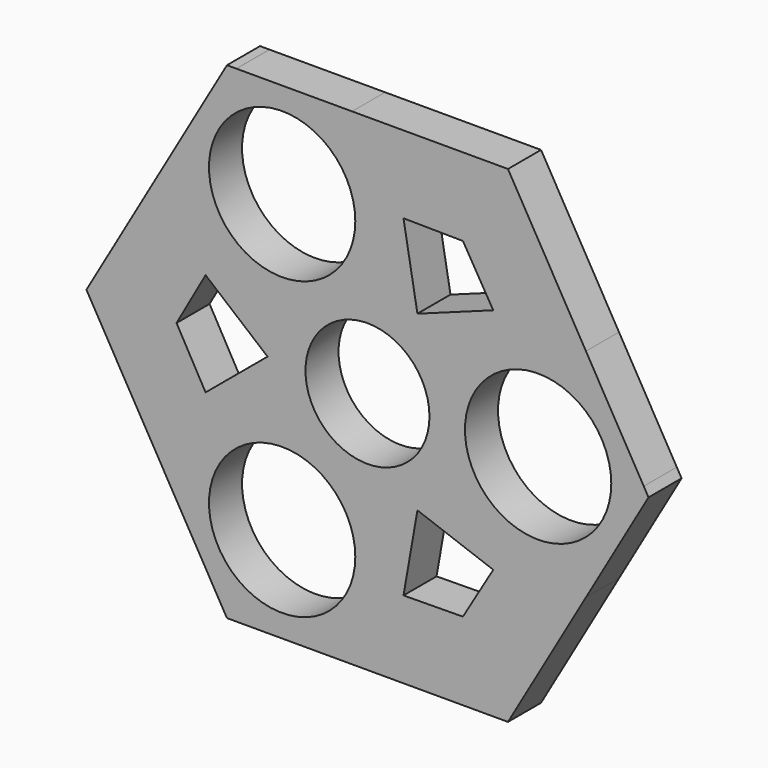
from build123d import *

# Parameters (mm, degrees)
F0_R     = 11.2395
F1_DEPTH = 6.35


# Not quite as in the source:
# - ends of sketch curves that miss each other by under 0.0002 mm in the source are joined


with BuildPart() as f1:
    # F0 (on Front) → F1 (new body)
    with BuildSketch(Plane.XZ):
        with BuildLine():
            Line((42.4466417494, 1.2702137502), (33.5675281941, 16.6492895541))
            Line((33.5675281941, 16.6492895541), (21.59, 37.3949769354))
            Line((21.59, 37.3949769354), (-2.3645964913, 37.3949769354))
            Line((-2.3645964913, 37.3949769354), (-20.1530883691, 37.3949769354))
            ThreePointArc((-20.1530883691, 37.3949769354), (-21.3957267903, 37.0536052726), (-22.3109030797, 36.1463361741))
            Line((-22.3109030797, 36.1463361741), (-31.2024712814, 20.7456882897))
            Line((-31.2024712814, 20.7456882897), (-43.18, 0))
            Line((-43.18, 0), (-31.2026751276, -20.7453352178))
            Line((-31.2026751276, -20.7453352178), (-22.3013335195, -36.1629111385))
            ThreePointArc((-22.3013335195, -36.1629111385), (-21.904358157, -36.6666327955), (-21.3938662061, -37.0548632868))
            ThreePointArc((-21.3938662061, -37.0548632868), (-20.7960911396, -37.3045921602), (-20.1545849957, -37.3949769354))
            Line((-20.1545849957, -37.3949769354), (-2.3645964913, -37.3949769354))
            Line((-2.3645964913, -37.3949769354), (21.59, -37.3949769354))
            Line((21.59, -37.3949769354), (33.5675281941, -16.6492895541))
            Line((33.5675281941, -16.6492895541), (42.4465800457, -1.269893127))
            Line((42.4465800457, -1.269893127), (42.4466570355, -1.2697597731))
            ThreePointArc((42.4466570355, -1.2697597731), (42.7869372237, 0.0002290365), (42.4466417494, 1.2702137502))
        make_face()
        with Locations((-13.1097560234, -22.7067635073)):
            Circle(F0_R, mode=Mode.SUBTRACT)
        Polygon((19.322999251, -17.547366104), (14.6677320258, -25.4052571005), (5.5348901331, -25.5078921242), (7.6610986638, -13.3857599047), (7.676716044, -13.2967206855), align=None, mode=Mode.SUBTRACT)
        Polygon((-15.3534299541, -0.0001902285), (-24.8221534826, -7.8882218978), (-24.8579644411, -7.9605251767), (-29.3354640516, 0), (-24.8579276431, 7.9605905996), (-24.8220816566, 7.8883561733), (-17.7474034479, 1.9942828585), align=None, mode=Mode.SUBTRACT)
        with Locations((-13.1097560234, 22.7067635073)):
            Circle(F0_R, mode=Mode.SUBTRACT)
        with BuildLine():
            ThreePointArc((-4.7625, 8.248891971), (4.7625, 8.248891971), (9.525, 0))
            ThreePointArc((9.525, 0), (-4.7625, -8.248891971), (-4.7625, 8.248891971))
        make_face(mode=Mode.SUBTRACT)
        with Locations((26.2195120463, 0.0001612286)):
            Circle(F0_R, mode=Mode.SUBTRACT)
        Polygon((5.5348901331, 25.5078921242), (14.6677320258, 25.4052571005), (19.322999251, 17.547366104), (7.676716044, 13.2967206855), (7.6610986638, 13.3857599047), align=None, mode=Mode.SUBTRACT)
        with BuildLine():
            Line((43.18, 0), (42.4466417494, 1.2702137502))
            ThreePointArc((42.4466417494, 1.2702137502), (42.7869372237, 0.0002290365), (42.4466570355, -1.2697597731))
            Line((42.4466570355, -1.2697597731), (42.4465800457, -1.269893127))
            Line((42.4465800457, -1.269893127), (33.5675281941, -16.6492895541))
            Line((33.5675281941, -16.6492895541), (43.18, 0))
        make_face()
        with BuildLine():
            Line((-20.1530883691, 37.3949769354), (-2.3645964913, 37.3949769354))
            Line((-2.3645964913, 37.3949769354), (-20.1235435545, 37.3951484857))
            ThreePointArc((-20.1235435545, 37.3951484857), (-20.1383162113, 37.3951056691), (-20.1530883691, 37.3949769354))
        make_face()
        with BuildLine():
            ThreePointArc((-22.3109030797, 36.1463361741), (-21.3957267903, 37.0536052726), (-20.1530883691, 37.3949769354))
            Line((-20.1530883691, 37.3949769354), (-21.59, 37.3949769354))
            Line((-21.59, 37.3949769354), (-22.3109030797, 36.1463361741))
        make_face()
        with BuildLine():
            Line((-31.2024712814, 20.7456882897), (-22.3109030797, 36.1463361741))
            ThreePointArc((-22.3109030797, 36.1463361741), (-22.3171177275, 36.1357499036), (-22.3232811402, 36.125133722))
            Line((-22.3232811402, 36.125133722), (-31.2024712814, 20.7456882897))
        make_face()
        with BuildLine():
            Line((-20.1238326592, -37.395162783), (-2.3645964913, -37.3949769354))
            Line((-2.3645964913, -37.3949769354), (-20.1545849957, -37.3949769354))
            ThreePointArc((-20.1545849957, -37.3949769354), (-20.1392091087, -37.3951164012), (-20.1238326592, -37.395162783))
        make_face()
        with BuildLine():
            Line((-21.59, -37.3949769354), (-20.1545849957, -37.3949769354))
            ThreePointArc((-20.1545849957, -37.3949769354), (-20.7960911396, -37.3045921602), (-21.3938662061, -37.0548632868))
            Line((-21.3938662061, -37.0548632868), (-21.590116174, -37.3947757161))
            Line((-21.590116174, -37.3947757161), (-21.59, -37.3949769354))
        make_face()
        with BuildLine():
            Line((-21.590116174, -37.3947757161), (-21.3938662061, -37.0548632868))
            ThreePointArc((-21.3938662061, -37.0548632868), (-21.904358157, -36.6666327955), (-22.3013335195, -36.1629111385))
            Line((-22.3013335195, -36.1629111385), (-21.590116174, -37.3947757161))
        make_face()
        with BuildLine():
            Line((-22.3013335195, -36.1629111385), (-31.2026751276, -20.7453352178))
            Line((-31.2026751276, -20.7453352178), (-22.3235850993, -36.1251258309))
            ThreePointArc((-22.3235850993, -36.1251258309), (-22.3125408514, -36.1440665044), (-22.3013335195, -36.1629111385))
        make_face()
    extrude(amount=F1_DEPTH)


solid = f1.part
